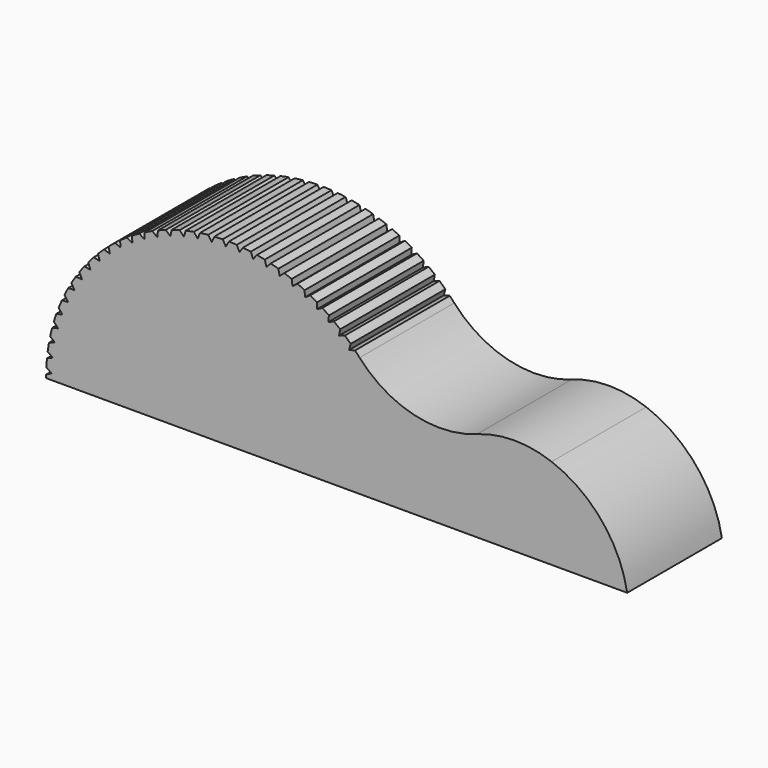
from build123d import *

# Parameters (mm, degrees)
F1_DEPTH         = 5.5
F3_DEPTH         = 5.501
F3_COPIES_COUNT  = 20
F3_COPIES_ANGLE  = 88.0004
F3_COPIES1_COUNT = 11
F3_COPIES1_ANGLE = 45


# Not quite as in the source:
# - a pattern or mirror of a feature is missing from the dataset's text; its kind, count and spacing are read off the source's solid


with BuildPart() as f1:
    # F0 (on Front) → F1 (new body)
    with BuildSketch(Plane.XZ):
        with BuildLine():
            Line((-27, 0), (0, 0))
            ThreePointArc((0, 0), (-1.1926360457, 2.5804184186), (-3.5143684573, 4.2206923475))
            ThreePointArc((-3.5143684573, 4.2206923475), (-5.2460959941, 4.5301572247), (-6.977823531, 4.2206923475))
            ThreePointArc((-6.977823531, 4.2206923475), (-9.9132769797, 4.0582856894), (-12.4325656492, 5.5736890919))
            ThreePointArc((-12.4325656492, 5.5736890919), (-21.6338668847, 7.7986561929), (-27, 0))
        make_face()
    extrude(amount=F1_DEPTH)

    # F2 (on face) → F3 (cut, through all)
    with BuildSketch(Plane.XZ.offset(5.5)):
        with BuildLine():
            ThreePointArc((-18.5063756326, 8.3487647015), (-18.65, 8.35), (-18.7936243674, 8.3487647015))
            Line((-18.7936243674, 8.3487647015), (-18.65, 8.1))
            Line((-18.65, 8.1), (-18.5063756326, 8.3487647015))
        make_face()
    f3 = extrude(amount=-F3_DEPTH, mode=Mode.SUBTRACT)

    # F3_copies: F3 ×20 about axis
    f3_copies_axis = Axis((-18.65, 0, 0), (0, -1, 0))
    for i in range(1, F3_COPIES_COUNT):
        add(f3.rotate(f3_copies_axis, i * F3_COPIES_ANGLE / (F3_COPIES_COUNT - 1)), mode=Mode.SUBTRACT)

    # F3_copies1: F3 ×11 about axis
    f3_copies1_axis = Axis((-18.65, 0, 0), (0, 1, 0))
    for i in range(1, F3_COPIES1_COUNT):
        add(f3.rotate(f3_copies1_axis, i * F3_COPIES1_ANGLE / (F3_COPIES1_COUNT - 1)), mode=Mode.SUBTRACT)


solid = f1.part
